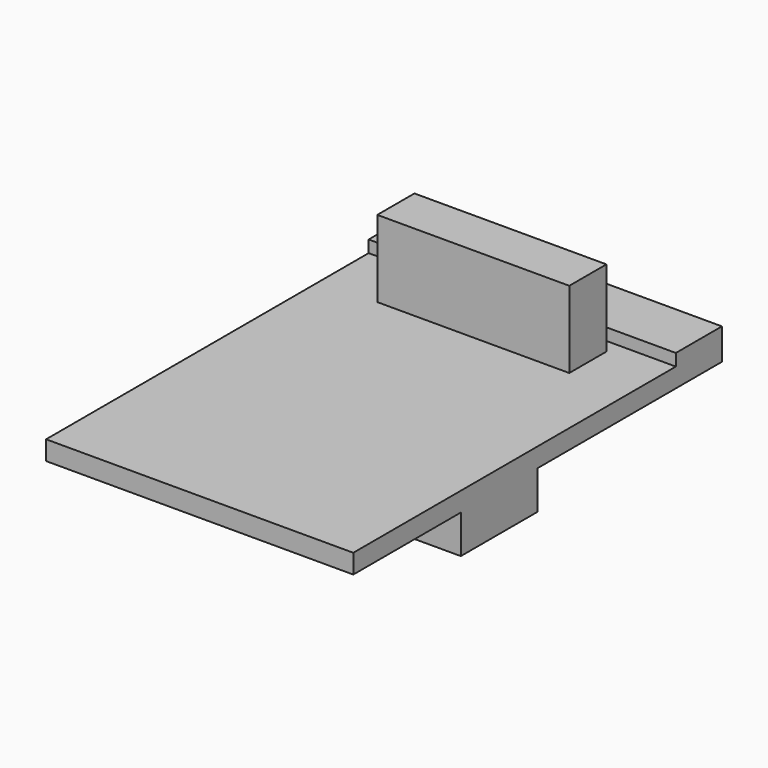
from build123d import *

# Parameters (mm, degrees)
F0_W     = 101.6
F0_H     = 152.4
F1_DEPTH = 6.35
F2_W     = 63.5
F2_H     = 15.3497201503
F3_DEPTH = 25.4
F4_W     = 101.6
F4_H     = 19.05
F5_DEPTH = 3.96875
F6_W     = 31.75
F6_H     = 31.75
F7_DEPTH = 12.7
F8_W     = 31.75
F8_H     = 31.75
F9_DEPTH = 12.7


# Not quite as in the source:
# - a length typed as a fraction of an inch, garbled in the dataset ("3 / 203.2 mm" for 3/8 in), is restored


with BuildPart() as f1:
    # F0 (on Top) → F1 (new body)
    with BuildSketch(Plane.XY):
        with Locations((50.8, 76.2)):
            Rectangle(F0_W, F0_H)
    extrude(amount=F1_DEPTH)

    # F2 (on face) → F3 (join)
    with BuildSketch(Plane.XY.offset(6.35)):
        with Locations((50.6108440459, 121.0213452578)):
            Rectangle(F2_W, F2_H)
    extrude(amount=F3_DEPTH)

    # F4 (on face) → F5 (join)
    with BuildSketch(Plane.XY.offset(6.35)):
        with Locations((50.8, 142.875)):
            Rectangle(F4_W, F4_H)
    extrude(amount=F5_DEPTH)

    # F6 (on face) → F7 (join)
    with BuildSketch(Plane(origin=(0, 0, 0), x_dir=(1, 0, 0), z_dir=(0, 0, -1))):
        with Locations((15.875, -60.3918848038)):
            Rectangle(F6_W, F6_H)
    extrude(amount=F7_DEPTH)

    # F8 (on face) → F9 (join)
    with BuildSketch(Plane(origin=(0, 0, 0), x_dir=(1, 0, 0), z_dir=(0, 0, -1))):
        with Locations((85.725, -60.325)):
            Rectangle(F8_W, F8_H)
    extrude(amount=F9_DEPTH)


solid = f1.part
